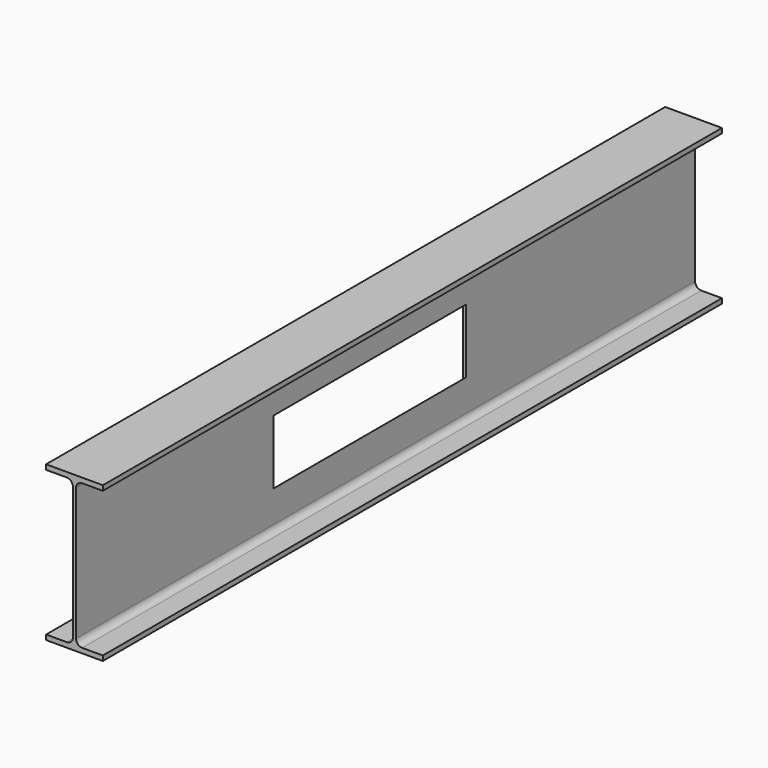
from build123d import *

# Parameters (mm, degrees)
F1_DEPTH      = 1500
F4_W          = 932.5531721115
F4_H          = 248.9361688495
F5_DEPTH      = 110.001
F5_DEPTH_BACK = 110.001
F6_SIZE       = 11.99999


# Not quite as in the source:
# - a fillet or chamfer is up to 0.001 mm smaller than in the source, because OpenCascade refuses the exact size
# - a feature of the source that left no trace in its solid (it failed there, or was rolled back) is left out


with BuildPart() as f1:
    # F0 (on Front) → F1 (new body, symmetric)
    with BuildSketch(Plane.XZ):
        with BuildLine():
            Line((110, 300), (-110, 300))
            Line((-110, 300), (-110, 281))
            Line((-110, 281), (-30, 281))
            ThreePointArc((-30, 281), (-13.0294372515, 273.9705627485), (-6, 257))
            Line((-6, 257), (-6, 0))
            Line((-6, 0), (-6, -257))
            ThreePointArc((-6, -257), (-13.0294372515, -273.9705627485), (-30, -281))
            Line((-30, -281), (-110, -281))
            Line((-110, -281), (-110, -300))
            Line((-110, -300), (110, -300))
            Line((110, -300), (110, -281))
            Line((110, -281), (30, -281))
            ThreePointArc((30, -281), (13.0294372515, -273.9705627485), (6, -257))
            Line((6, -257), (6, 0))
            Line((6, 0), (6, 257))
            ThreePointArc((6, 257), (13.0294372515, 273.9705627485), (30, 281))
            Line((30, 281), (110, 281))
            Line((110, 281), (110, 300))
        make_face()
    extrude(amount=F1_DEPTH, both=True)

    # F4 (on Right) → F5 (cut, two sides)
    with BuildSketch(Plane.YZ) as f5_sk:
        with Locations((-75.63829422, -9.5744766295)):
            Rectangle(F4_W, F4_H)
    extrude(amount=-F5_DEPTH, mode=Mode.SUBTRACT)
    extrude(f5_sk.sketch, amount=F5_DEPTH_BACK, mode=Mode.SUBTRACT)

    # F6 (size 12 in the source; OpenCascade refuses exactly that, so slightly less here)
    f6_edges = [f1.edges().sort_by_distance(p)[0] for p in [
        (-6, -75.638294, 114.893608),
        (-6, -75.638294, -134.042561),
    ]]
    chamfer(f6_edges, length=F6_SIZE)


solid = f1.part
